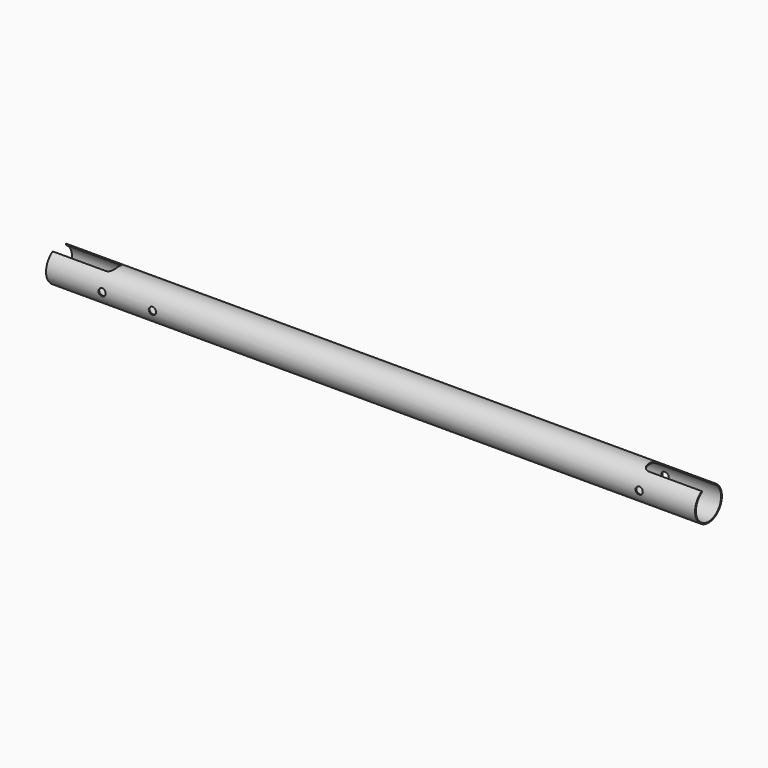
from build123d import *

# Parameters (mm, degrees)
F0_R          = 19.05
F0_R_2        = 17.8689
F1_DEPTH      = 368.3
F2_R          = 4.1275
F3_DEPTH      = 19.051
F3_DEPTH_BACK = 19.051
F4_W          = 82.55
F4_H          = 19.05
F5_DEPTH      = 19.0510001
F6_T4_DEPTH   = 33.1291873733
F6_S5_R       = 19.05
F6_T6_DEPTH   = 19
F6_S7_R       = 17.8689
F6_T8_DEPTH   = 19
F6_T12_DEPTH  = 33.1291873733
F6_S13_R      = 19.05
F6_T14_DEPTH  = 19
F6_S15_R      = 17.8689
F6_T16_DEPTH  = 19
F6_T20_DEPTH  = 33.1291873733
F6_S21_R      = 19.05
F6_T22_DEPTH  = 19
F6_S23_R      = 17.8689
F6_T24_DEPTH  = 19
F6_T28_DEPTH  = 33.1291873733
F6_S29_R      = 19.05
F6_T30_DEPTH  = 19
F6_S31_R      = 17.8689
F6_T32_DEPTH  = 19


# Not quite as in the source:
# - a fillet or chamfer that OpenCascade refuses, or shapes differently, is made with other operations: its cross-section is extruded or revolved along the edge and cut away or added


with BuildPart() as f1:
    # F0 (on Right) → F1 (new body, symmetric)
    with BuildSketch(Plane.YZ):
        Circle(F0_R)
        Circle(F0_R_2, mode=Mode.SUBTRACT)
    extrude(amount=F1_DEPTH, both=True)

    # F2 (on Front) → F3 (cut, two sides)
    with BuildSketch(Plane.XZ) as f3_sk:
        with Locations((-304.8, 0)):
            Circle(F2_R)
        with Locations((304.8, 0)):
            Circle(F2_R)
        with Locations((-247.65, 0)):
            Circle(F2_R)
    extrude(amount=-F3_DEPTH, mode=Mode.SUBTRACT)
    extrude(f3_sk.sketch, amount=F3_DEPTH_BACK, mode=Mode.SUBTRACT)

    # F4 (on Top) → F5 (cut, through all)
    with BuildSketch(Plane.XY):
        with Locations((-342.9, 0)):
            Rectangle(F4_W, F4_H)
        with Locations((342.9, 0)):
            Rectangle(F4_W, F4_H)
    extrude(amount=F5_DEPTH, mode=Mode.SUBTRACT)

    # F6: fillet of radius 6.35 on 4 edges, made by hand


with BuildPart() as f6_tool2:
    # F6_s3 → F6_t4 (new body)
    with BuildSketch(Plane.XY.offset(-0.7564034312)):
        with BuildLine():
            ThreePointArc((-301.625, 3.175), (-303.4848719395, 7.6651280605), (-307.975, 9.525))
            Line((-307.975, 9.525), (-301.625, 9.525))
            Line((-301.625, 9.525), (-301.625, 3.175))
        make_face()
    extrude(amount=F6_T4_DEPTH)

    # F6_s5 → F6_t6 (intersect, symmetric)
    with BuildSketch(Plane.YZ.offset(-304.8)):
        Circle(F6_S5_R)
    extrude(amount=F6_T6_DEPTH, both=True, mode=Mode.INTERSECT)

    # F6_s7 → F6_t8 (cut, symmetric)
    with BuildSketch(Plane.YZ.offset(-304.8)):
        Circle(F6_S7_R)
    extrude(amount=F6_T8_DEPTH, both=True, mode=Mode.SUBTRACT)


with BuildPart() as f1_1:
    add(f1.part)

    # F6_t1: union F6_tool2
    add(f6_tool2.part)


with BuildPart() as f6_tool10:
    # F6_s11 → F6_t12 (new body)
    with BuildSketch(Plane.XY.offset(-0.7564034312)):
        with BuildLine():
            ThreePointArc((-307.975, -9.525), (-303.4848719395, -7.6651280605), (-301.625, -3.175))
            Line((-301.625, -3.175), (-301.625, -9.525))
            Line((-301.625, -9.525), (-307.975, -9.525))
        make_face()
    extrude(amount=F6_T12_DEPTH)

    # F6_s13 → F6_t14 (intersect, symmetric)
    with BuildSketch(Plane.YZ.offset(-304.8)):
        Circle(F6_S13_R)
    extrude(amount=F6_T14_DEPTH, both=True, mode=Mode.INTERSECT)

    # F6_s15 → F6_t16 (cut, symmetric)
    with BuildSketch(Plane.YZ.offset(-304.8)):
        Circle(F6_S15_R)
    extrude(amount=F6_T16_DEPTH, both=True, mode=Mode.SUBTRACT)


with BuildPart() as f1_2:
    add(f1_1.part)

    # F6_t9: union F6_tool10
    add(f6_tool10.part)


with BuildPart() as f6_tool18:
    # F6_s19 → F6_t20 (new body)
    with BuildSketch(Plane.XY.offset(-0.7564034312)):
        with BuildLine():
            ThreePointArc((307.975, 9.525), (303.4848719395, 7.6651280605), (301.625, 3.175))
            Line((301.625, 3.175), (301.625, 9.525))
            Line((301.625, 9.525), (307.975, 9.525))
        make_face()
    extrude(amount=F6_T20_DEPTH)

    # F6_s21 → F6_t22 (intersect, symmetric)
    with BuildSketch(Plane.YZ.offset(304.8)):
        Circle(F6_S21_R)
    extrude(amount=F6_T22_DEPTH, both=True, mode=Mode.INTERSECT)

    # F6_s23 → F6_t24 (cut, symmetric)
    with BuildSketch(Plane.YZ.offset(304.8)):
        Circle(F6_S23_R)
    extrude(amount=F6_T24_DEPTH, both=True, mode=Mode.SUBTRACT)


with BuildPart() as f1_3:
    add(f1_2.part)

    # F6_t17: union F6_tool18
    add(f6_tool18.part)


with BuildPart() as f6_tool26:
    # F6_s27 → F6_t28 (new body)
    with BuildSketch(Plane.XY.offset(-0.7564034312)):
        with BuildLine():
            ThreePointArc((301.625, -3.175), (303.4848719395, -7.6651280605), (307.975, -9.525))
            Line((307.975, -9.525), (301.625, -9.525))
            Line((301.625, -9.525), (301.625, -3.175))
        make_face()
    extrude(amount=F6_T28_DEPTH)

    # F6_s29 → F6_t30 (intersect, symmetric)
    with BuildSketch(Plane.YZ.offset(304.8)):
        Circle(F6_S29_R)
    extrude(amount=F6_T30_DEPTH, both=True, mode=Mode.INTERSECT)

    # F6_s31 → F6_t32 (cut, symmetric)
    with BuildSketch(Plane.YZ.offset(304.8)):
        Circle(F6_S31_R)
    extrude(amount=F6_T32_DEPTH, both=True, mode=Mode.SUBTRACT)


with BuildPart() as f1_4:
    add(f1_3.part)

    # F6_t25: union F6_tool26
    add(f6_tool26.part)


solid = f1_4.part
